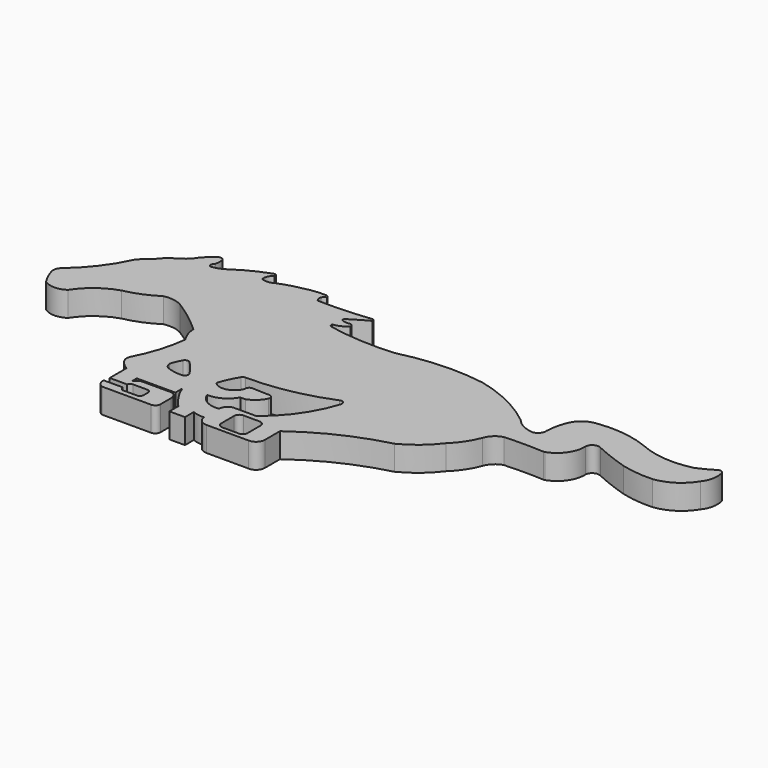
from build123d import *

# Parameters (mm, degrees)
F0_W     = 1.5955208801
F0_H     = 1.1417223141
F1_DEPTH = 2.54
F2_R     = 0.381


# Not quite as in the source:
# - a feature names something its author has since deleted; it is built from what else it names


with BuildPart() as f1:
    # F0 (on Top) → F1 (new body)
    with BuildSketch(Plane.XY):
        with BuildLine():
            ThreePointArc((-17.853555356, 8.3740441176), (-17.797850048, 9.0234844386), (-17.9735293317, 9.6511886693))
            ThreePointArc((-17.9735293317, 9.6511886693), (-18.7702044575, 9.095594444), (-19.4845060376, 8.437453538))
            ThreePointArc((-19.4845060376, 8.437453538), (-20.0769728416, 7.6889871), (-20.8468619562, 7.1246382062))
            ThreePointArc((-20.8468619562, 7.1246382062), (-21.5535932044, 6.6397751602), (-22.1349055344, 6.0099837619))
            ThreePointArc((-22.1349055344, 6.0099837619), (-22.8020037999, 5.4653402422), (-23.373411446, 4.821018924))
            ThreePointArc((-23.373411446, 4.821018924), (-24.9570436982, 2.2101334539), (-27.0641564536, 0))
            ThreePointArc((-27.0641564536, 0), (-27.3013792374, -0.4059980502), (-27.3118564678, -0.8761036698))
            ThreePointArc((-27.3118564678, -0.8761036698), (-26.9762696426, -1.7588388711), (-26.5192129181, -2.585240168))
            ThreePointArc((-26.5192129181, -2.585240168), (-25.3797891537, -2.9473127207), (-24.2403653893, -2.585240168))
            ThreePointArc((-24.2403653893, -2.585240168), (-22.7687501944, -0.9970956803), (-20.8468619562, 0))
            ThreePointArc((-20.8468619562, 0), (-19.1618737041, 0.5114383216), (-17.6019793103, 1.3284352904))
            ThreePointArc((-17.6019793103, 1.3284352904), (-16.6114613748, 1.3658120585), (-15.6699110228, 1.0559641311))
            ThreePointArc((-15.6699110228, 1.0559641311), (-13.836990045, -0.2128519809), (-12.1277868024, -1.6439766827))
            ThreePointArc((-12.1277868024, -1.6439766827), (-11.9336363035, -2.596456984), (-11.5065968044, -3.4696983061))
            ThreePointArc((-11.5065968044, -3.4696983061), (-12.0603763693, -6.1074027488), (-13.0972628465, -8.5951774506))
            ThreePointArc((-13.0972628465, -8.5951774506), (-13.1571271668, -8.9304230164), (-13.0972628465, -9.2656685821))
            ThreePointArc((-13.0972628465, -9.2656685821), (-12.6673723448, -9.8597669968), (-12.0776668191, -10.2956639603))
            Line((-12.0776668191, -10.2956639603), (-6.3745881725, -10.2815440897))
            ThreePointArc((-6.3745881725, -10.2815440897), (-5.661175229, -11.6523680947), (-4.7017061152, -12.8637868911))
            Line((-4.7017061152, -12.8637868911), (-3.1061852351, -12.8637868911))
            ThreePointArc((-3.1061852351, -12.8637868911), (-2.5046193085, -13.0450341984), (-1.8773153965, -13.0799906328))
            Line((-1.8773153965, -13.0799906328), (-1.8773153965, -11.1498029349))
            ThreePointArc((-1.8773153965, -11.1498029349), (-3.2358026465, -10.9194336675), (-4.1321902536, -9.8729887977))
            ThreePointArc((-4.1321902536, -9.8729887977), (-2.762101982, -9.5557238553), (-1.7820949775, -8.5470687176))
            ThreePointArc((-1.7820949775, -8.5470687176), (-1.5222103345, -8.563510241), (-1.2623256915, -8.5470687176))
            ThreePointArc((-1.2623256915, -8.5470687176), (-0.2521144999, -7.8636169747), (0.296981619, -6.7745226773))
            ThreePointArc((0.296981619, -6.7745226773), (-1.0695443684, -6.7459053087), (-2.4351383708, -6.6878945441))
            ThreePointArc((-2.4351383708, -6.6878945441), (-2.47662666, -7.3075469995), (-2.8703414029, -7.7878376875))
            ThreePointArc((-2.8703414029, -7.7878376875), (-3.8634480384, -8.215930963), (-4.8555368558, -7.7854841948))
            ThreePointArc((-4.8555368558, -7.7854841948), (-4.4118591918, -6.6546279705), (-3.8211325325, -5.5931536733))
            ThreePointArc((-3.8211325325, -5.5931536733), (0.9463155332, -5.1460447662), (5.4981125468, -3.6595686038))
            ThreePointArc((5.4981125468, -3.6595686038), (3.9292310446, -7.3247476474), (1.2548560917, -10.2815440897))
            Line((1.2548560917, -10.2815440897), (3.424389055, -10.2815440897))
            ThreePointArc((3.424389055, -10.2815440897), (4.0684620951, -10.5312307256), (4.3759387918, -11.1498029349))
            ThreePointArc((4.3759387918, -11.1498029349), (8.4470385599, -8.7170246357), (12.9095430064, -7.1113105765))
            ThreePointArc((12.9095430064, -7.1113105765), (14.6499014784, -5.9750044202), (16.0797765196, -4.4665294757))
            ThreePointArc((16.0797765196, -4.4665294757), (17.0824134117, -3.2848508213), (17.7962558926, -1.9093239797))
            ThreePointArc((17.7962558926, -1.9093239797), (18.2693374956, -1.158544739), (19.0398292625, -0.7182969583))
            ThreePointArc((19.0398292625, -0.7182969583), (21.1040388769, -0.6580801248), (23.1682484913, -0.7182969583))
            ThreePointArc((23.1682484913, -0.7182969583), (24.6618788785, 0.3509323406), (25.1962952316, 2.1083685951))
            ThreePointArc((25.1962952316, 2.1083685951), (25.5625360075, 2.688610955), (26.2486916035, 2.686610911))
            ThreePointArc((26.2486916035, 2.686610911), (27.9563627814, 1.9695236008), (29.7065656632, 1.3635987416))
            ThreePointArc((29.7065656632, 1.3635987416), (31.3072851011, 1.0747081226), (32.9331687986, 1.0271401629))
            ThreePointArc((32.9331687986, 1.0271401629), (34.8022907173, 1.7067846532), (36.1881435322, 3.1332997622))
            ThreePointArc((36.1881435322, 3.1332997622), (36.6947166808, 4.4258458038), (36.4090675868, 5.7844098323))
            ThreePointArc((36.4090675868, 5.7844098323), (35.3773820938, 5.1441520424), (34.2787277468, 4.6271765887))
            ThreePointArc((34.2787277468, 4.6271765887), (31.4645162229, 4.4186578639), (28.7347726999, 5.1340366859))
            ThreePointArc((28.7347726999, 5.1340366859), (26.1330502463, 5.8052334102), (23.4462247687, 5.7844098323))
            ThreePointArc((23.4462247687, 5.7844098323), (22.2537986567, 5.3443509735), (21.4882896661, 4.3296944714))
            ThreePointArc((21.4882896661, 4.3296944714), (21.1738764805, 3.3083388634), (21.0508802065, 2.2467858285))
            ThreePointArc((21.0508802065, 2.2467858285), (20.8743202019, 1.6656557288), (20.3426897543, 1.3719642325))
            ThreePointArc((20.3426897543, 1.3719642325), (19.1770408937, 1.6925240778), (18.2389527963, 2.4550767658))
            ThreePointArc((18.2389527963, 2.4550767658), (15.213228604, 4.3764336471), (11.8444237953, 5.6002691403))
            ThreePointArc((11.8444237953, 5.6002691403), (7.4617172468, 5.8553669147), (3.1170349339, 5.2253453558))
            ThreePointArc((3.1170349339, 5.2253453558), (-0.3222546999, 5.1769365744), (-3.7357347618, 5.6002691403))
            ThreePointArc((-3.7357347618, 5.6002691403), (-3.9109790902, 5.7380499014), (-3.9648547442, 5.954363393))
            ThreePointArc((-3.9648547442, 5.954363393), (-3.2076855094, 6.1579091097), (-2.5662026437, 6.6087259705))
            ThreePointArc((-2.5662026437, 6.6087259705), (-2.6816745227, 6.8506790556), (-2.9344122405, 6.9401144859))
            ThreePointArc((-2.9344122405, 6.9401144859), (-3.3411836345, 6.9201756162), (-3.7357347618, 7.0211208162))
            ThreePointArc((-3.7357347618, 7.0211208162), (-3.7991866915, 7.2149721455), (-3.6634675098, 7.3672376669))
            ThreePointArc((-3.6634675098, 7.3672376669), (-2.7399402466, 7.9339930521), (-1.7939161675, 8.4623420981))
            ThreePointArc((-1.7939161675, 8.4623420981), (-1.8199119342, 8.6408630831), (-1.9853852552, 8.7127247699))
            ThreePointArc((-1.9853852552, 8.7127247699), (-4.6980995714, 8.4860922136), (-7.4201607773, 8.4623420981))
            ThreePointArc((-7.4201607773, 8.4623420981), (-7.5947711332, 8.7475985275), (-7.5674446161, 9.0809350967))
            ThreePointArc((-7.5674446161, 9.0809350967), (-7.4270233398, 9.2667316603), (-7.2139635978, 9.3607744389))
            ThreePointArc((-7.2139635978, 9.3607744389), (-7.3278655543, 9.5771146023), (-7.5674446161, 9.6258854459))
            ThreePointArc((-7.5674446161, 9.6258854459), (-8.6833589555, 9.5799434946), (-9.7785029647, 9.3607744389))
            ThreePointArc((-9.7785029647, 9.3607744389), (-10.8930573942, 9.0992536146), (-11.9706566565, 8.7127247699))
            ThreePointArc((-11.9706566565, 8.7127247699), (-12.5959752787, 8.5066336569), (-13.2463167914, 8.6093606885))
            ThreePointArc((-13.2463167914, 8.6093606885), (-13.2014829624, 9.1909284241), (-12.8128398197, 9.6258854459))
            ThreePointArc((-12.8128398197, 9.6258854459), (-12.8828043149, 9.8816424228), (-13.1472356177, 9.9012063658))
            ThreePointArc((-13.1472356177, 9.9012063658), (-14.9102034334, 9.1429725714), (-16.5531244409, 8.1511134234))
            ThreePointArc((-16.5531244409, 8.1511134234), (-17.1785091382, 7.8557594105), (-17.853555356, 7.7052515483))
            ThreePointArc((-17.853555356, 7.7052515483), (-18.0466206726, 7.8917547722), (-17.9774053631, 8.1511134234))
            ThreePointArc((-17.9774053631, 8.1511134234), (-17.8804815168, 8.2431350284), (-17.853555356, 8.3740441176))
        make_face()
        with BuildLine():
            ThreePointArc((-9.8634943458, -7.5188701169), (-9.5759120441, -6.726862178), (-9.1238332832, -6.0158031442))
            ThreePointArc((-9.1238332832, -6.0158031442), (-8.0815611968, -7.1046448545), (-7.2634754698, -8.3706002705))
            ThreePointArc((-7.2634754698, -8.3706002705), (-8.3889522856, -8.4455851495), (-9.4824567107, -8.1688743492))
            ThreePointArc((-9.4824567107, -8.1688743492), (-9.7629961953, -7.8966430618), (-9.8634943458, -7.5188701169))
        make_face(mode=Mode.SUBTRACT)
        with BuildLine():
            Line((-6.3745881725, -10.2815440897), (-12.0776668191, -10.2956639603))
            Line((-12.0776668191, -10.2956639603), (-12.0776668191, -12.4645475298))
            Line((-12.0776668191, -12.4645475298), (-10.2948714048, -12.4645475298))
            ThreePointArc((-10.2948714048, -12.4645475298), (-10.151821337, -12.250239437), (-9.9078435451, -12.1673773974))
            Line((-9.9078435451, -12.1673773974), (-8.4426673129, -12.1673773974))
            ThreePointArc((-8.4426673129, -12.1673773974), (-8.1903544086, -12.2545634175), (-8.0832848325, -12.4991023913))
            Line((-8.0832848325, -12.4991023913), (-8.0832848325, -13.0865313113))
            ThreePointArc((-8.0832848325, -13.0865313113), (-8.1760539897, -13.3627931009), (-8.4426673129, -13.480453752))
            Line((-8.4426673129, -13.480453752), (-9.9285766482, -13.480453752))
            ThreePointArc((-9.9285766482, -13.480453752), (-10.1420812696, -13.3214733755), (-10.2672260255, -13.0865313113))
            Line((-10.2672260255, -13.0865313113), (-12.1885407716, -13.0865313113))
            ThreePointArc((-12.1885407716, -13.0865313113), (-12.0698333288, -13.6464984914), (-11.6356443614, -14.0195060521))
            Line((-11.6356443614, -14.0195060521), (-6.5626808431, -14.0195060521))
            ThreePointArc((-6.5626808431, -14.0195060521), (-6.1877507829, -13.858338598), (-6.0338711055, -13.4803590442))
            Line((-6.0338711055, -13.4803590442), (-6.0372729786, -12.10632734))
            ThreePointArc((-6.0372729786, -12.10632734), (-6.1863238807, -11.639008832), (-6.5626808431, -11.324432615))
            Line((-6.5626808431, -11.324432615), (-9.7416797653, -11.3323032856))
            ThreePointArc((-9.7416797653, -11.3323032856), (-10.0816695519, -11.495017768), (-10.3345368552, -11.7745301733))
            Line((-10.3345368552, -11.7745301733), (-10.3360521158, -11.1625096717))
            Line((-10.3360521158, -11.1625096717), (-6.3724313448, -11.1526964084))
            Line((-6.3724313448, -11.1526964084), (-6.3745881725, -10.2815440897))
        make_face()
        with Locations((-3.9039456751, -13.4346480481)):
            Rectangle(F0_W, F0_H)
        with BuildLine():
            Line((-1.8773153965, -11.1498029349), (-1.8773153965, -13.0799906328))
            ThreePointArc((-1.8773153965, -13.0799906328), (-1.5774509554, -13.7273078382), (-0.9146768716, -13.9912562445))
            Line((-0.9146768716, -13.9912562445), (3.424389055, -13.9912562445))
            ThreePointArc((3.424389055, -13.9912562445), (4.0946903926, -13.7387492982), (4.3759387918, -13.0799906328))
            Line((4.3759387918, -13.0799906328), (4.3759387918, -11.1498029349))
            ThreePointArc((4.3759387918, -11.1498029349), (4.0684620951, -10.5312307256), (3.424389055, -10.2815440897))
            Line((3.424389055, -10.2815440897), (1.2548560917, -10.2815440897))
            Line((1.2548560917, -10.2815440897), (-0.9146768716, -10.2815440897))
            ThreePointArc((-0.9146768716, -10.2815440897), (-1.5837154327, -10.5075491381), (-1.8773153965, -11.1498029349))
        make_face()
        with BuildLine():
            Line((0.3667430137, -10.8470208943), (1.2548560917, -10.8470208943))
            Line((1.2548560917, -10.8470208943), (2.155655995, -10.8470208943))
            ThreePointArc((2.155655995, -10.8470208943), (2.4447859495, -11.060725144), (2.5549547281, -11.4029655233))
            Line((2.5549547281, -11.4029655233), (2.5549547281, -13.0613548681))
            ThreePointArc((2.5549547281, -13.0613548681), (2.44161419, -13.369377396), (2.155655995, -13.5304732248))
            Line((2.155655995, -13.5304732248), (0.3667430137, -13.5304732248))
            ThreePointArc((0.3667430137, -13.5304732248), (0.0242937564, -13.403738151), (-0.153145098, -13.0846006796))
            Line((-0.153145098, -13.0846006796), (-0.153145098, -11.4029655233))
            ThreePointArc((-0.153145098, -11.4029655233), (-0.0138348624, -11.012183253), (0.3667430137, -10.8470208943))
        make_face(mode=Mode.SUBTRACT)
    extrude(amount=F1_DEPTH)

    # F2
    f2_edges = [f1.edges().sort_by_distance(p)[0] for p in [
        (-17.973529, 9.651189, 1.27),
        (-2.435138, -6.687895, 1.27),
        (0.296982, -6.774523, 1.27),
        (5.498113, -3.659569, 1.27),
        (-3.821133, -5.593154, 1.27),
        (-9.123833, -6.015803, 1.27),
        (-7.263475, -8.3706, 1.27),
        (36.409068, 5.78441, 1.27),
        (23.168248, -0.718297, 1.27),
    ]]
    fillet(f2_edges, radius=F2_R)


solid = f1.part
